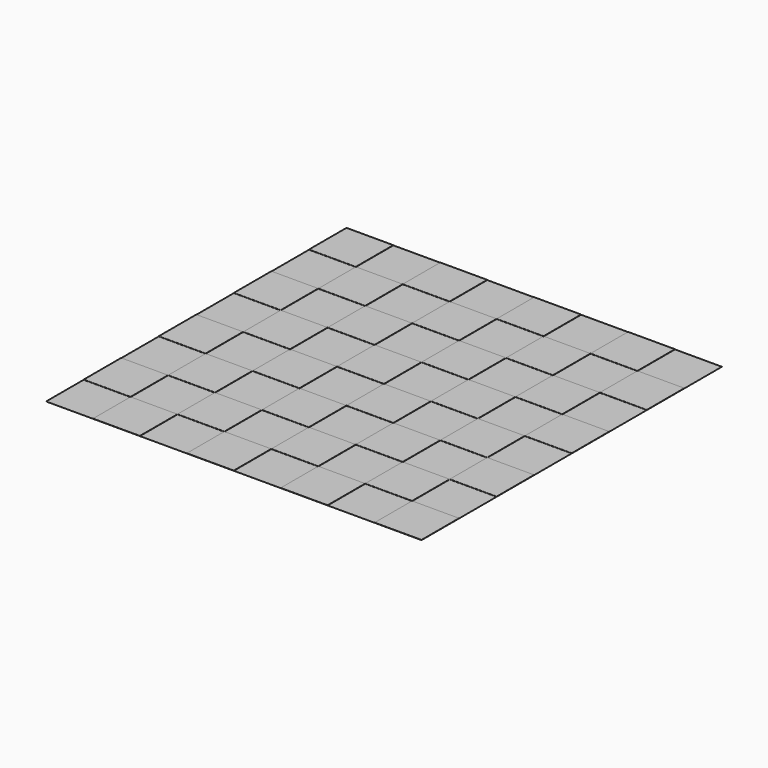
from build123d import *

# Parameters (mm, degrees)
F0_W     = 31.6957823275
F0_H     = 31.75
F1_DEPTH = 0.127
F0_W_2   = 31.75
F2_W     = 127
F2_H     = 254
F3_DEPTH = 0.00254
F4_W     = 127
F4_H     = 254
F5_DEPTH = 0.00254


with BuildPart() as f1:
    # F0 (on Top) → F1 (new body)
    with BuildSketch(Plane.XY):
        with Locations((-88.7057874083, 156.3674052)):
            Rectangle(F0_W, F0_H)
    extrude(amount=F1_DEPTH)


with BuildPart() as f1b:
    # F0 (on Top) → F1, piece 2 (new body)
    with BuildSketch(Plane.XY):
        with Locations((-56.9557874083, 124.6174052)):
            Rectangle(F0_W, F0_H)
    extrude(amount=F1_DEPTH)


with BuildPart() as f1c:
    # F0 (on Top) → F1, piece 3 (new body)
    with BuildSketch(Plane.XY):
        with Locations((-25.2328962445, 156.3674052)):
            Rectangle(F0_W_2, F0_H)
    extrude(amount=F1_DEPTH)


with BuildPart() as f1d:
    # F0 (on Top) → F1, piece 4 (new body)
    with BuildSketch(Plane.XY):
        with Locations((6.5171037555, 124.6174052)):
            Rectangle(F0_W_2, F0_H)
    extrude(amount=F1_DEPTH)


with BuildPart() as f1e:
    # F0 (on Top) → F1, piece 5 (new body)
    with BuildSketch(Plane.XY):
        with Locations((38.2671037555, 156.3674052)):
            Rectangle(F0_W_2, F0_H)
    extrude(amount=F1_DEPTH)


with BuildPart() as f1f:
    # F0 (on Top) → F1, piece 6 (new body)
    with BuildSketch(Plane.XY):
        with Locations((70.0171037555, 124.6174052)):
            Rectangle(F0_W_2, F0_H)
    extrude(amount=F1_DEPTH)


with BuildPart() as f1g:
    # F0 (on Top) → F1, piece 7 (new body)
    with BuildSketch(Plane.XY):
        with Locations((101.7671037555, 156.3674052)):
            Rectangle(F0_W_2, F0_H)
    extrude(amount=F1_DEPTH)


with BuildPart() as f1h:
    # F0 (on Top) → F1, piece 8 (new body)
    with BuildSketch(Plane.XY):
        with Locations((133.5171037555, 124.6174052)):
            Rectangle(F0_W_2, F0_H)
    extrude(amount=F1_DEPTH)


with BuildPart() as f1i:
    # F0 (on Top) → F1, piece 9 (new body)
    with BuildSketch(Plane.XY):
        with Locations((101.7671037555, 92.8674052)):
            Rectangle(F0_W_2, F0_H)
    extrude(amount=F1_DEPTH)


with BuildPart() as f1j:
    # F0 (on Top) → F1, piece 10 (new body)
    with BuildSketch(Plane.XY):
        with Locations((70.0171037555, 61.1174052)):
            Rectangle(F0_W_2, F0_H)
    extrude(amount=F1_DEPTH)


with BuildPart() as f1k:
    # F0 (on Top) → F1, piece 11 (new body)
    with BuildSketch(Plane.XY):
        with Locations((38.2671037555, 92.8674052)):
            Rectangle(F0_W_2, F0_H)
    extrude(amount=F1_DEPTH)


with BuildPart() as f1l:
    # F0 (on Top) → F1, piece 12 (new body)
    with BuildSketch(Plane.XY):
        with Locations((6.5171037555, 61.1174052)):
            Rectangle(F0_W_2, F0_H)
    extrude(amount=F1_DEPTH)


with BuildPart() as f1m:
    # F0 (on Top) → F1, piece 13 (new body)
    with BuildSketch(Plane.XY):
        with Locations((-25.2328962445, 92.8674052)):
            Rectangle(F0_W_2, F0_H)
    extrude(amount=F1_DEPTH)


with BuildPart() as f1n:
    # F0 (on Top) → F1, piece 14 (new body)
    with BuildSketch(Plane.XY):
        with Locations((-56.9557874083, 61.1174052)):
            Rectangle(F0_W, F0_H)
    extrude(amount=F1_DEPTH)


with BuildPart() as f1o:
    # F0 (on Top) → F1, piece 15 (new body)
    with BuildSketch(Plane.XY):
        with Locations((-88.7057874083, 92.8674052)):
            Rectangle(F0_W, F0_H)
    extrude(amount=F1_DEPTH)


with BuildPart() as f1p:
    # F0 (on Top) → F1, piece 16 (new body)
    with BuildSketch(Plane.XY):
        with Locations((-88.7057874083, 29.3674052)):
            Rectangle(F0_W, F0_H)
    extrude(amount=F1_DEPTH)


with BuildPart() as f1q:
    # F0 (on Top) → F1, piece 17 (new body)
    with BuildSketch(Plane.XY):
        with Locations((-56.9557874083, -2.3825948)):
            Rectangle(F0_W, F0_H)
    extrude(amount=F1_DEPTH)


with BuildPart() as f1r:
    # F0 (on Top) → F1, piece 18 (new body)
    with BuildSketch(Plane.XY):
        with Locations((-25.2328962445, 29.3674052)):
            Rectangle(F0_W_2, F0_H)
    extrude(amount=F1_DEPTH)


with BuildPart() as f1s:
    # F0 (on Top) → F1, piece 19 (new body)
    with BuildSketch(Plane.XY):
        with Locations((6.5171037555, -2.3825948)):
            Rectangle(F0_W_2, F0_H)
    extrude(amount=F1_DEPTH)


with BuildPart() as f1t:
    # F0 (on Top) → F1, piece 20 (new body)
    with BuildSketch(Plane.XY):
        with Locations((38.2671037555, 29.3674052)):
            Rectangle(F0_W_2, F0_H)
    extrude(amount=F1_DEPTH)


with BuildPart() as f1u:
    # F0 (on Top) → F1, piece 21 (new body)
    with BuildSketch(Plane.XY):
        with Locations((70.0171037555, -2.3825948)):
            Rectangle(F0_W_2, F0_H)
    extrude(amount=F1_DEPTH)


with BuildPart() as f1v:
    # F0 (on Top) → F1, piece 22 (new body)
    with BuildSketch(Plane.XY):
        with Locations((101.7671037555, 29.3674052)):
            Rectangle(F0_W_2, F0_H)
    extrude(amount=F1_DEPTH)


with BuildPart() as f1w:
    # F0 (on Top) → F1, piece 23 (new body)
    with BuildSketch(Plane.XY):
        with Locations((133.5171037555, -2.3825948)):
            Rectangle(F0_W_2, F0_H)
    extrude(amount=F1_DEPTH)


with BuildPart() as f1x:
    # F0 (on Top) → F1, piece 24 (new body)
    with BuildSketch(Plane.XY):
        with Locations((133.5171037555, 61.1174052)):
            Rectangle(F0_W_2, F0_H)
    extrude(amount=F1_DEPTH)


with BuildPart() as f1y:
    # F0 (on Top) → F1, piece 25 (new body)
    with BuildSketch(Plane.XY):
        with Locations((-88.7057874083, -34.1325948)):
            Rectangle(F0_W, F0_H)
    extrude(amount=F1_DEPTH)


with BuildPart() as f1z:
    # F0 (on Top) → F1, piece 26 (new body)
    with BuildSketch(Plane.XY):
        with Locations((-56.9557874083, -65.8825948)):
            Rectangle(F0_W, F0_H)
    extrude(amount=F1_DEPTH)


with BuildPart() as f1ba:
    # F0 (on Top) → F1, piece 27 (new body)
    with BuildSketch(Plane.XY):
        with Locations((-25.2328962445, -34.1325948)):
            Rectangle(F0_W_2, F0_H)
    extrude(amount=F1_DEPTH)


with BuildPart() as f1bb:
    # F0 (on Top) → F1, piece 28 (new body)
    with BuildSketch(Plane.XY):
        with Locations((6.5171037555, -65.8825948)):
            Rectangle(F0_W_2, F0_H)
    extrude(amount=F1_DEPTH)


with BuildPart() as f1bc:
    # F0 (on Top) → F1, piece 29 (new body)
    with BuildSketch(Plane.XY):
        with Locations((70.0171037555, -65.8825948)):
            Rectangle(F0_W_2, F0_H)
    extrude(amount=F1_DEPTH)


with BuildPart() as f1bd:
    # F0 (on Top) → F1, piece 30 (new body)
    with BuildSketch(Plane.XY):
        with Locations((133.5171037555, -65.8825948)):
            Rectangle(F0_W_2, F0_H)
    extrude(amount=F1_DEPTH)


with BuildPart() as f1be:
    # F0 (on Top) → F1, piece 31 (new body)
    with BuildSketch(Plane.XY):
        with Locations((38.2671037555, -34.1325948)):
            Rectangle(F0_W_2, F0_H)
    extrude(amount=F1_DEPTH)


with BuildPart() as f1bf:
    # F0 (on Top) → F1, piece 32 (new body)
    with BuildSketch(Plane.XY):
        with Locations((101.7671037555, -34.1325948)):
            Rectangle(F0_W_2, F0_H)
    extrude(amount=F1_DEPTH)


with BuildPart() as f3:
    # F2 (on Top) → F3 (new body)
    with BuildSketch(Plane.XY):
        with Locations((85.8921037555, 45.2424052)):
            Rectangle(F2_W, F2_H)
    extrude(amount=-F3_DEPTH)


with BuildPart() as f5:
    # F4 (on Top) → F5 (new body)
    with BuildSketch(Plane.XY):
        with Locations((-41.0536785721, 45.2424052)):
            Rectangle(F4_W, F4_H)
    extrude(amount=-F5_DEPTH)


solid = Compound([f1.part, f1b.part, f1c.part, f1d.part, f1e.part, f1f.part, f1g.part, f1h.part, f1i.part, f1j.part, f1k.part, f1l.part, f1m.part, f1n.part, f1o.part, f1p.part, f1q.part, f1r.part, f1s.part, f1t.part, f1u.part, f1v.part, f1w.part, f1x.part, f1y.part, f1z.part, f1ba.part, f1bb.part, f1bc.part, f1bd.part, f1be.part, f1bf.part, f3.part, f5.part])
